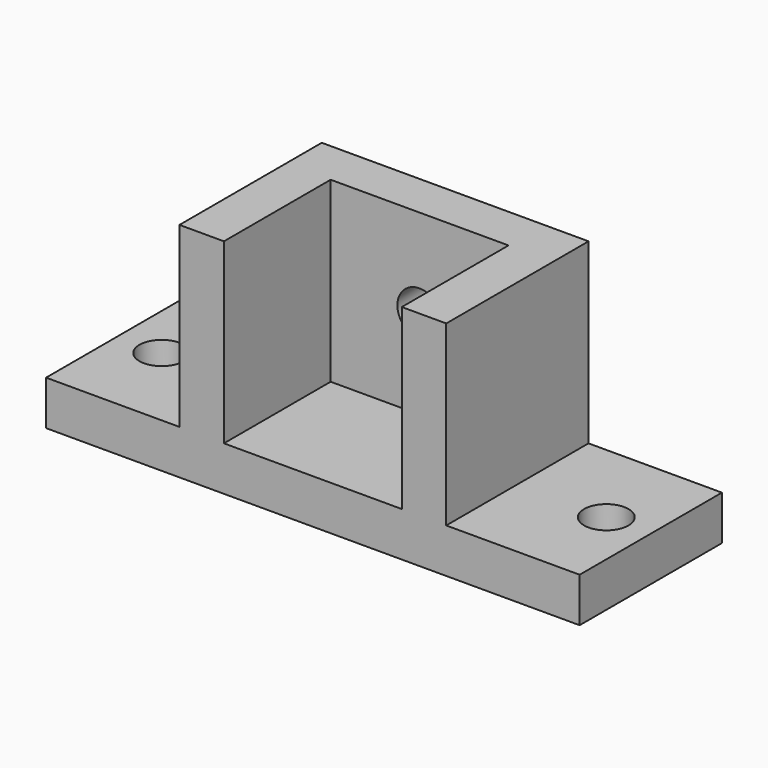
from build123d import *

# Parameters (mm, degrees)
F0_W     = 60
F0_H     = 20
F1_DEPTH = 5
F3_DEPTH = 20
F5_D     = 5
F7_D     = 5


# Not quite as in the source:
# - a pattern or mirror of a feature is missing from the dataset's text; its kind, count and spacing are read off the source's solid


with BuildPart() as f1:
    # F0 (on Top) → F1 (new body)
    with BuildSketch(Plane.XY):
        Rectangle(F0_W, F0_H)
    extrude(amount=F1_DEPTH)

    # F2 (on face) → F3 (join)
    with BuildSketch(Plane.XY.offset(5)):
        Polygon((-15, 10), (-15, -10), (-10, -10), (-10, 5), (0, 5), (0, 10), align=None)
    f3 = extrude(amount=F3_DEPTH)

    # F3_copies: F3 across plane
    add(f3.mirror(Plane(origin=(0, 0, 0), x_dir=(0, 0, 1), z_dir=(1, 0, 0))))

    # F5 (through all)
    with Locations(Plane.XY.offset(5)):
        with Locations((-25, 0)):
            f5 = Hole(F5_D / 2)

    # F5_copies: F5 across plane
    add(f5.mirror(Plane(origin=(0, 0, 0), x_dir=(0, 0, 1), z_dir=(1, 0, 0))), mode=Mode.SUBTRACT)

    # F7 (through all)
    with Locations(Plane.XZ.offset(-5)):
        with Locations((0, 15)):
            Hole(F7_D / 2)


solid = f1.part
